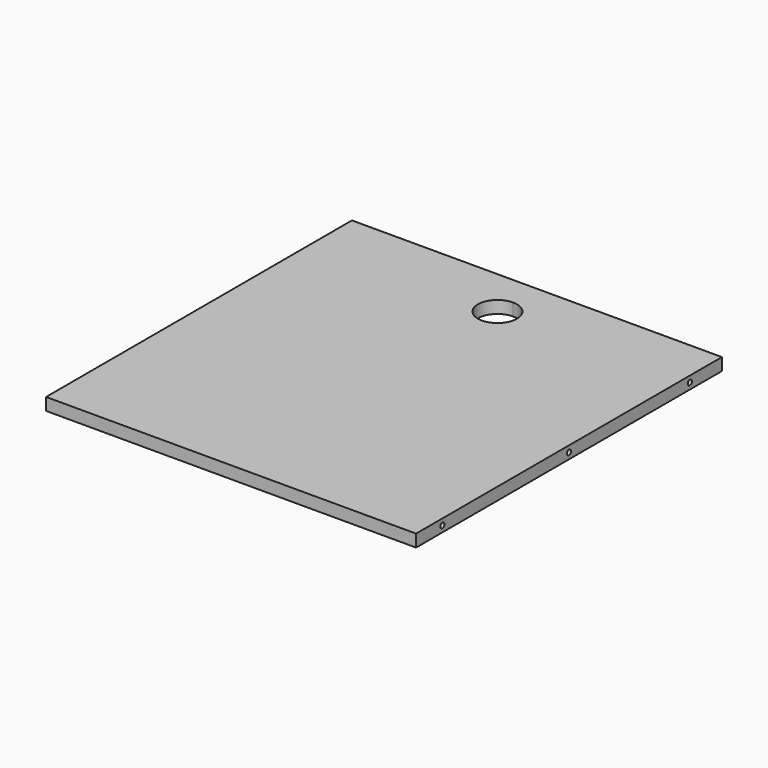
from build123d import *

# Parameters (mm, degrees)
F1_DEPTH = 19.05
F3_D     = 15.0114
F3_DEPTH = 14.224
F3_TIP   = 4.5098795482
F5_D     = 8.001
F5_DEPTH = 25.4
F5_TIP   = 2.4037429064
F7_D     = 8.001
F7_DEPTH = 25.4
F7_TIP   = 2.4037429064


# Not quite as in the source:
# - a feature names something its author has since deleted; it is built from what else it names


with BuildPart() as f1:
    # F0 (on Top) → F1 (new body)
    with BuildSketch(Plane.XY):
        Polygon((285.75, -295.275), (285.75, 295.275), (0, 295.275), (-285.75, 295.275), (-285.75, -295.275), align=None)
        with BuildLine():
            ThreePointArc((30.1625, 219.075), (-21.3281082875, 197.7468917125), (0, 249.2375))
            ThreePointArc((0, 249.2375), (21.3281082875, 240.4031082875), (30.1625, 219.075))
        make_face(mode=Mode.SUBTRACT)
    extrude(amount=F1_DEPTH)

    # F3
    with Locations(Plane(origin=(0, 0, 0), x_dir=(1, 0, 0), z_dir=(0, 0, -1))):
        with Locations((-261.874, 244.475), (261.874, 244.475), (-261.874, 0), (261.874, 0), (261.874, -244.475), (-261.874, -244.475)):
            Hole(F3_D / 2, depth=F3_DEPTH)
            with Locations((0, 0, -(F3_DEPTH + F3_TIP / 2))):  # 118° drill point
                Cone(0, F3_D / 2, F3_TIP, mode=Mode.SUBTRACT)

    # F5
    with Locations(Plane.YZ.offset(285.75)):
        with Locations((-244.475, 9.525), (0, 9.525), (233.3625, 9.525)):
            Hole(F5_D / 2, depth=F5_DEPTH)
            with Locations((0, 0, -(F5_DEPTH + F5_TIP / 2))):  # 118° drill point
                Cone(0, F5_D / 2, F5_TIP, mode=Mode.SUBTRACT)

    # F7
    with Locations(Plane(origin=(-285.75, 0, 0), x_dir=(0, -1, 0), z_dir=(-1, 0, 0))):
        with Locations((0, 9.525), (244.475, 9.525), (-244.475, 9.525)):
            Hole(F7_D / 2, depth=F7_DEPTH)
            with Locations((0, 0, -(F7_DEPTH + F7_TIP / 2))):  # 118° drill point
                Cone(0, F7_D / 2, F7_TIP, mode=Mode.SUBTRACT)


solid = f1.part
